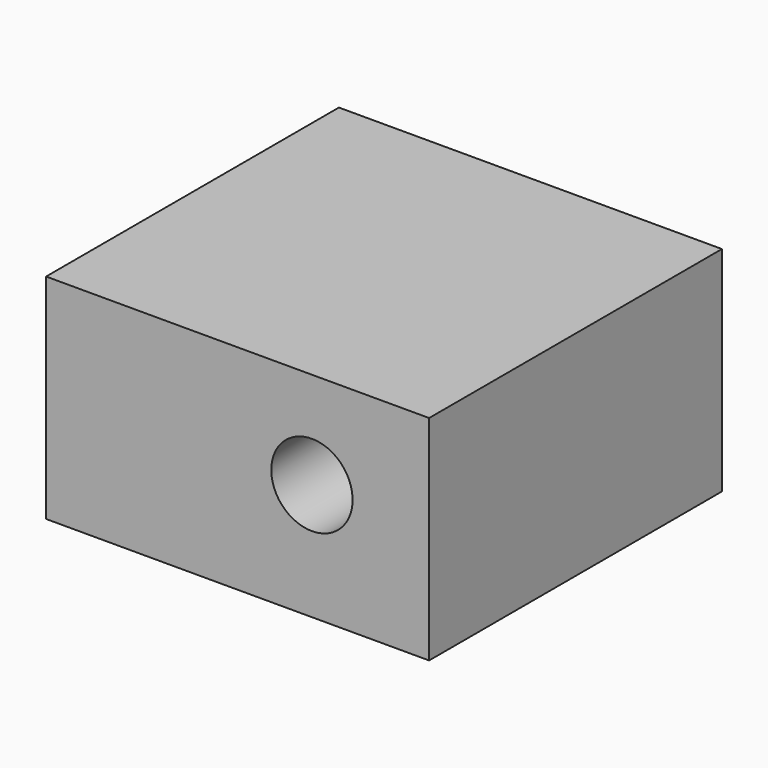
from build123d import *

# Parameters (mm, degrees)
F0_W     = 94.1855311394
F0_H     = 52.4866655469
F1_DEPTH = 90
F4_D     = 20
F4_DEPTH = 80
F4_TIP   = 6.0086061903
F5_R     = 9.112196694
F7_DEPTH = 80


# Not quite as in the source:
# - the program builds the solid bodies; features that only make, move or delete a surface that nothing else refers to are left out


with BuildPart() as f1:
    # F0 (on Front) → F1 (new body)
    with BuildSketch(Plane.XZ):
        with Locations((9.957909584, -2.3857913911)):
            Rectangle(F0_W, F0_H)
    extrude(amount=F1_DEPTH)

    # F4
    with Locations(Plane.XZ.offset(90)):
        with Locations((28.2388776541, 0)):
            Hole(F4_D / 2, depth=F4_DEPTH)
            with Locations((0, 0, -(F4_DEPTH + F4_TIP / 2))):  # 118° drill point
                Cone(0, F4_D / 2, F4_TIP, mode=Mode.SUBTRACT)

    # F5 (on face) → F7 (cut)
    with BuildSketch(Plane.XZ.offset(90)):
        with Locations((-17.2343160957, 0)):
            Circle(F5_R)
    extrude(amount=F7_DEPTH, mode=Mode.SUBTRACT)


solid = f1.part
